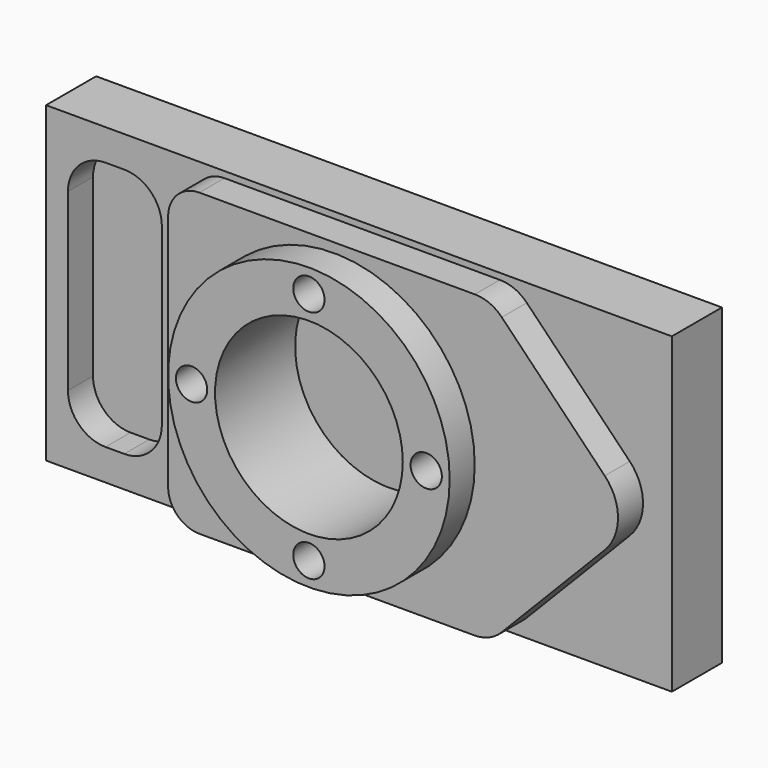
from build123d import *

# Parameters (mm, degrees)
F0_W      = 200
F0_H      = 100
F1_DEPTH  = 20
F3_DEPTH  = 10
F5_DEPTH  = 10
F6_R      = 45
F7_DEPTH  = 10
F8_R      = 30
F9_DEPTH  = 32
F11_D     = 10
F11_DEPTH = 15
F11_TIP   = 3.0043030951


# Not quite as in the source:
# - a feature names something its author has since deleted; it is built from what else it names


with BuildPart() as f1:
    # F0 (on Front) → F1 (new body)
    with BuildSketch(Plane.XZ):
        Rectangle(F0_W, F0_H)
    extrude(amount=F1_DEPTH)

    # F2 (on face) → F3 (cut)
    with BuildSketch(Plane.XZ.offset(20)):
        with BuildLine():
            Line((-75, 40), (-81, 40))
            ThreePointArc((-81, 40), (-89.4852813742, 36.4852813742), (-93, 28))
            Line((-93, 28), (-93, -28))
            ThreePointArc((-93, -28), (-89.4852813742, -36.4852813742), (-81, -40))
            Line((-81, -40), (-75, -40))
            ThreePointArc((-75, -40), (-66.5147186258, -36.4852813742), (-63, -28))
            Line((-63, -28), (-63, 28))
            ThreePointArc((-63, 28), (-66.5147186258, 36.4852813742), (-75, 40))
        make_face()
    extrude(amount=-F3_DEPTH, mode=Mode.SUBTRACT)

    # F4 (on face) → F5 (join)
    with BuildSketch(Plane.XZ.offset(20)):
        with BuildLine():
            Line((45.028, 48), (-43, 48))
            ThreePointArc((-43, 48), (-50.0710678119, 45.0710678119), (-53, 38))
            Line((-53, 38), (-53, -38))
            ThreePointArc((-53, -38), (-50.0710678119, -45.0710678119), (-43, -48))
            Line((-43, -48), (45.028, -48))
            ThreePointArc((45.028, -48), (49.6343185527, -47.0344012956), (53.515, -44.3715338615))
            Line((53.515, -44.3715338615), (86.5275302355, -10.4637753147))
            ThreePointArc((86.5275302355, -10.4637753147), (90.7799947329, -0.0125702902), (86.5450528262, 10.4457473475))
            Line((86.5450528262, 10.4457473475), (53.640042261, 44.356597878))
            ThreePointArc((53.640042261, 44.356597878), (49.7035120288, 47.0516780295), (45.028, 48))
        make_face()
    extrude(amount=F5_DEPTH)

    # F6 (on face) → F7 (join)
    with BuildSketch(Plane.XZ.offset(30)):
        Circle(F6_R)
    extrude(amount=F7_DEPTH)

    # F8 (on face) → F9 (cut)
    with BuildSketch(Plane.XZ.offset(40)):
        Circle(F8_R)
    extrude(amount=-F9_DEPTH, mode=Mode.SUBTRACT)

    # F11
    with Locations(Plane.XZ.offset(40)):
        with Locations((-37.5, 0), (0, 37.5), (37.5, 0), (0, -37.5)):
            Hole(F11_D / 2, depth=F11_DEPTH)
            with Locations((0, 0, -(F11_DEPTH + F11_TIP / 2))):  # 118° drill point
                Cone(0, F11_D / 2, F11_TIP, mode=Mode.SUBTRACT)


solid = f1.part
